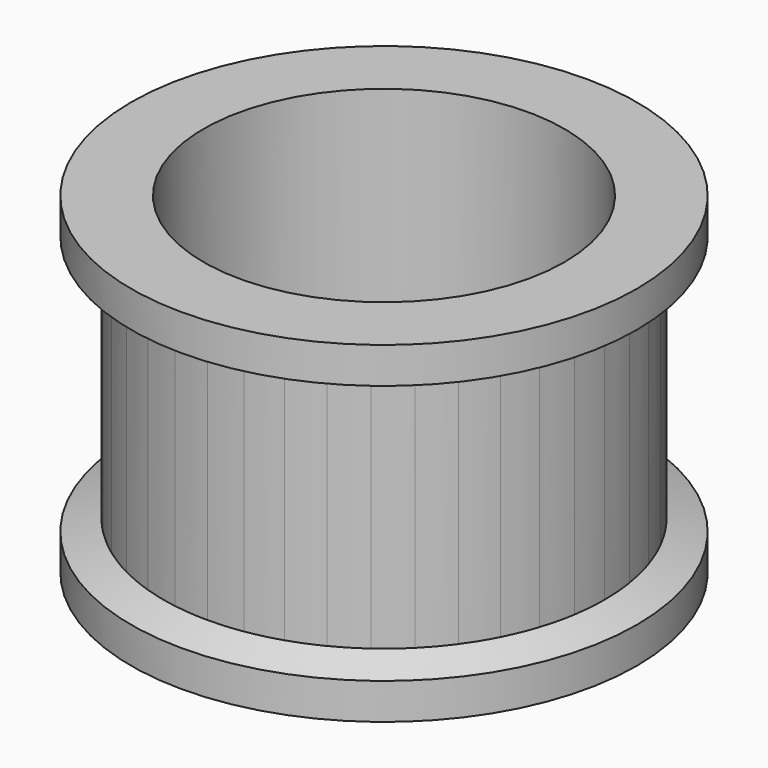
from build123d import *

# Parameters (mm, degrees)
F3_DEPTH = 4.5
F4_COUNT = 20
F7_R     = 5
F8_DEPTH = 50


# Not quite as in the source:
# - a feature names something its author has since deleted; it is built from what else it names


with BuildPart() as f3:
    # F2 (on Top) → F3 (new body, symmetric)
    with BuildSketch(Plane.XY):
        with BuildLine():
            Line((0.8388325323, 5.2961801716), (0.9561583811, 6.0369464271))
            ThreePointArc((0.9561583811, 6.0369464271), (0.4795575063, 6.0933558579), (0, 6.1121977237))
            ThreePointArc((0, 6.1121977237), (-0.2034624056, 6.108810364), (-0.4066992948, 6.0986520393))
            ThreePointArc((-0.4066992948, 6.0986520393), (-0.682126936, 6.074015464), (-0.9561583811, 6.0369464271))
            Line((-0.9561583811, 6.0369464271), (-0.8388325323, 5.2961801716))
            Line((-0.8388325323, 5.2961801716), (0, 0))
            Line((0, 0), (0.8388325323, 5.2961801716))
        make_face()
    extrude(amount=F3_DEPTH, both=True)

    # F4: F3 ×20 about axis
    f4_axis = Axis((0, 0, 0), (0, 0, -1))


with BuildPart() as f3_1:
    add(f3.part)
    for i in range(1, F4_COUNT):
        add(f3.part.rotate(f4_axis, i * 360 / F4_COUNT))

    # F5 (on Front) → F6 (revolve)
    with BuildSketch(Plane.XZ):
        Polygon((7.002817496, 4.5), (0, 4.5), (0, 2.9028632371), (5.3621977237, 2.9028632371), (7.002817496, 3.5), align=None)
        Polygon((5.3621977237, -3.0971367629), (0, -3.0971367629), (0, -4.6942735258), (7.002817496, -4.6942735258), (7.002817496, -3.6942735258), align=None)
    revolve(axis=Axis((0, 0, 3.7014316186), (0, 0, 1)))

    # F7 (on Top) → F8 (cut, symmetric)
    with BuildSketch(Plane.XY):
        Circle(F7_R)
    extrude(amount=F8_DEPTH, both=True, mode=Mode.SUBTRACT)


solid = f3_1.part
